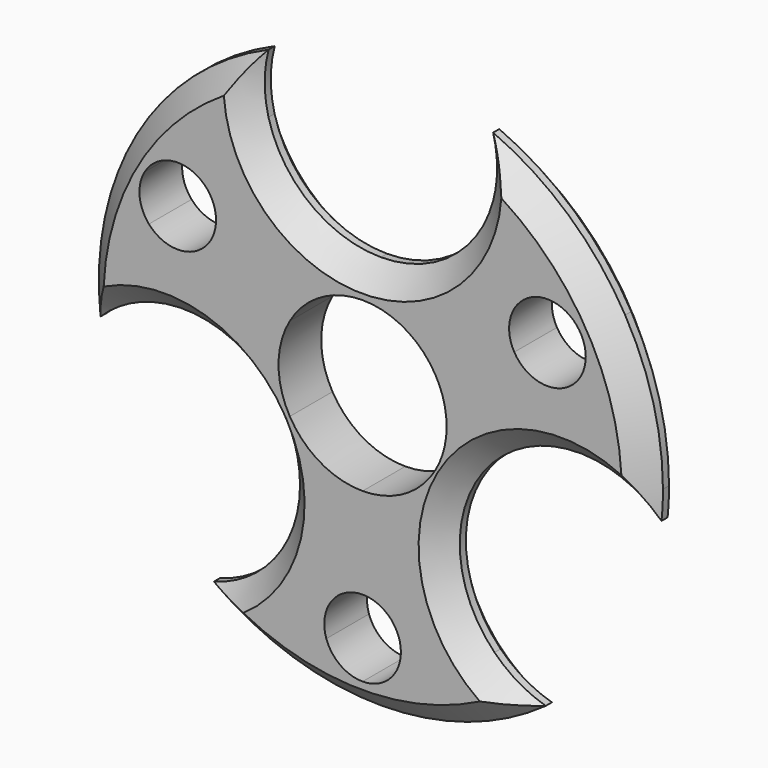
from build123d import *

# Parameters (mm, degrees)
F1_DEPTH     = 7
F2_T2_ANGLE  = 96.7405372454
F2_T4_ANGLE  = 266.8582437325
F2_T6_ANGLE  = 95.969109219
F2_T8_ANGLE  = 264.3512540772
F2_T10_ANGLE = 268.0965177518
F2_T12_ANGLE = 96.2209043171
F2_T14_ANGLE = 96.2209043171
F2_T16_ANGLE = 264.3512540772
F2_T18_ANGLE = 95.969109219
F2_T20_ANGLE = 266.8582437325
F2_T22_ANGLE = 96.7405372454
F2_T24_ANGLE = 268.0965177518


# Not quite as in the source:
# - a fillet or chamfer that OpenCascade refuses, or shapes differently, is made with other operations: its cross-section is extruded or revolved along the edge and cut away or added


with BuildPart() as f1:
    # F0 (on Front) → F1 (new body)
    with BuildSketch(Plane.XZ):
        with BuildLine():
            Line((-28.60048896, 16.5125), (-32.04293994, 18.5))
            ThreePointArc((-32.04293994, 18.5), (-36.2110940276, 7.5997808734), (-36.7769641036, -4.0564653732))
            ThreePointArc((-36.7769641036, -4.0564653732), (-33.6399342951, -1.6712337769), (-29.9995629467, -0.1619351868))
            ThreePointArc((-29.9995629467, -0.1619351868), (-29.5180509711, 5.3558068364), (-28.030388979, 10.6909912395))
            ThreePointArc((-28.030388979, 10.6909912395), (-29.2497876853, 13.5102449097), (-28.60048896, 16.5125))
        make_face()
        with BuildLine():
            ThreePointArc((-28.030388979, 10.6909912395), (-29.5180509711, 5.3558068364), (-29.9995629467, -0.1619351868))
            ThreePointArc((-29.9995629467, -0.1619351868), (-20.1170678219, -0.7895806962), (-12.6676409298, -7.3136659008))
            Line((-12.6676409298, -7.3136659008), (-9.5479300767, -5.5125))
            ThreePointArc((-9.5479300767, -5.5125), (-11.025, 0), (-9.5479300767, 5.5125))
            Line((-9.5479300767, 5.5125), (-19.8969336519, 11.4875))
            ThreePointArc((-19.8969336519, 11.4875), (-23.7589562157, 8.9989236207), (-28.030388979, 10.6909912395))
        make_face()
        with BuildLine():
            ThreePointArc((0, 14.7547752324), (-9.310283358, 17.9279039927), (-14.7448970108, 26.1263853631))
            ThreePointArc((-14.7448970108, 26.1263853631), (-19.3469694385, 22.9280346638), (-23.2738644946, 18.9295333141))
            ThreePointArc((-23.2738644946, 18.9295333141), (-20.3661071395, 17.1899858756), (-19.223711306, 14))
            ThreePointArc((-19.223711306, 14), (-19.3949340289, 12.6994342984), (-19.8969336519, 11.4875))
            Line((-19.8969336519, 11.4875), (-9.5479300767, 5.5125))
            ThreePointArc((-9.5479300767, 5.5125), (-5.5125, 9.5479300767), (0, 11.025))
            Line((0, 11.025), (0, 14.7547752324))
        make_face()
        with BuildLine():
            ThreePointArc((-14.7448970108, 26.1263853631), (-15.2451824532, 30.0359191128), (-14.726480194, 33.9430520298))
            ThreePointArc((-14.726480194, 33.9430520298), (-24.6265431784, 27.6140067915), (-32.04293994, 18.5))
            Line((-32.04293994, 18.5), (-28.60048896, 16.5125))
            ThreePointArc((-28.60048896, 16.5125), (-26.3251091458, 18.5759367359), (-23.2738644946, 18.9295333141))
            ThreePointArc((-23.2738644946, 18.9295333141), (-19.3469694385, 22.9280346638), (-14.7448970108, 26.1263853631))
        make_face()
        with BuildLine():
            ThreePointArc((19.8969336519, 11.4875), (19.6727745701, 16.0763978398), (23.2738644946, 18.9295333141))
            ThreePointArc((23.2738644946, 18.9295333141), (19.3469694385, 22.9280346638), (14.7448970108, 26.1263853631))
            ThreePointArc((14.7448970108, 26.1263853631), (9.310283358, 17.9279039927), (0, 14.7547752324))
            Line((0, 14.7547752324), (0, 11.025))
            ThreePointArc((0, 11.025), (5.5125, 9.5479300767), (9.5479300767, 5.5125))
            Line((9.5479300767, 5.5125), (19.8969336519, 11.4875))
        make_face()
        with BuildLine():
            Line((28.60048896, 16.5125), (32.04293994, 18.5))
            ThreePointArc((32.04293994, 18.5), (24.6265431784, 27.6140067915), (14.726480194, 33.9430520298))
            ThreePointArc((14.726480194, 33.9430520298), (15.1149822826, 31.9885142218), (15.2452247676, 30))
            ThreePointArc((15.2452247676, 30), (15.1196254471, 28.0471035473), (14.7448970108, 26.1263853631))
            ThreePointArc((14.7448970108, 26.1263853631), (19.3469694385, 22.9280346638), (23.2738644946, 18.9295333141))
            ThreePointArc((23.2738644946, 18.9295333141), (26.3251091458, 18.5759367359), (28.60048896, 16.5125))
        make_face()
        with BuildLine():
            ThreePointArc((36.8122346311, -3.7228190211), (36.9530288431, -1.8637755563), (37, 0))
            ThreePointArc((37, 0), (35.7392555727, 9.5763046688), (32.04293994, 18.5))
            Line((32.04293994, 18.5), (28.60048896, 16.5125))
            ThreePointArc((28.60048896, 16.5125), (29.1024885831, 15.3005657016), (29.273711306, 14))
            ThreePointArc((29.273711306, 14), (28.9526221952, 12.2325590968), (28.030388979, 10.6909912395))
            ThreePointArc((28.030388979, 10.6909912395), (29.4933804082, 5.4900375314), (29.9997945679, 0.1110219992))
            ThreePointArc((29.9997945679, 0.1110219992), (33.6494620505, -1.3733111503), (36.8122346311, -3.7228190211))
        make_face()
        with BuildLine():
            ThreePointArc((12.4392811828, -7.1818223394), (19.983625223, -0.5594336383), (29.9997945679, 0.1110219992))
            ThreePointArc((29.9997945679, 0.1110219992), (29.4933804082, 5.4900375314), (28.030388979, 10.6909912395))
            ThreePointArc((28.030388979, 10.6909912395), (23.7589562157, 8.9989236207), (19.8969336519, 11.4875))
            Line((19.8969336519, 11.4875), (9.5479300767, 5.5125))
            ThreePointArc((9.5479300767, 5.5125), (10.6493322348, 2.8534799723), (11.025, 0))
            ThreePointArc((11.025, 0), (10.6493322348, -2.8534799723), (9.5479300767, -5.5125))
            Line((9.5479300767, -5.5125), (12.4392811828, -7.1818223394))
        make_face()
        with BuildLine():
            ThreePointArc((4.7565244845, -29.6205245536), (9.9921782342, -28.2870354427), (14.9037494122, -26.0360952037))
            ThreePointArc((14.9037494122, -26.0360952037), (10.476296354, -17.0266102837), (12.4392811828, -7.1818223394))
            Line((12.4392811828, -7.1818223394), (9.5479300767, -5.5125))
            ThreePointArc((9.5479300767, -5.5125), (5.5125, -9.5479300767), (0, -11.025))
            Line((0, -11.025), (0, -22.975))
            ThreePointArc((0, -22.975), (3.5532115755, -24.4467884245), (5.025, -28))
            ThreePointArc((5.025, -28), (4.9574267788, -28.8213067227), (4.7565244845, -29.6205245536))
        make_face()
        with BuildLine():
            ThreePointArc((-10.6080939152, -15), (-11.7862202639, -20.9020258568), (-15.1400214589, -25.8994160209))
            ThreePointArc((-15.1400214589, -25.8994160209), (-10.1207607074, -28.2412854294), (-4.7565244845, -29.6205245536))
            ThreePointArc((-4.7565244845, -29.6205245536), (-4.0861816456, -25.0753214605), (0, -22.975))
            Line((0, -22.975), (0, -11.025))
            ThreePointArc((0, -11.025), (-5.5125, -9.5479300767), (-9.5479300767, -5.5125))
            Line((-9.5479300767, -5.5125), (-12.6676409298, -7.3136659008))
            ThreePointArc((-12.6676409298, -7.3136659008), (-11.1319048818, -11.0212606962), (-10.6080939152, -15))
        make_face()
        with BuildLine():
            ThreePointArc((-21.9014841146, -29.8215525011), (-11.5239437142, -35.1596177634), (0, -37))
            Line((0, -37), (0, -33.025))
            ThreePointArc((0, -33.025), (-2.9246785395, -32.0861816456), (-4.7565244845, -29.6205245536))
            ThreePointArc((-4.7565244845, -29.6205245536), (-10.1207607074, -28.2412854294), (-15.1400214589, -25.8994160209))
            ThreePointArc((-15.1400214589, -25.8994160209), (-18.267298054, -28.2974207927), (-21.9014841146, -29.8215525011))
        make_face()
        with BuildLine():
            ThreePointArc((0, -37), (11.3644165831, -35.2115043093), (21.6301731615, -30.0189208501))
            ThreePointArc((21.6301731615, -30.0189208501), (18.0140533687, -28.4546333842), (14.9037494122, -26.0360952037))
            ThreePointArc((14.9037494122, -26.0360952037), (9.9921782342, -28.2870354427), (4.7565244845, -29.6205245536))
            ThreePointArc((4.7565244845, -29.6205245536), (2.9246785395, -32.0861816456), (0, -33.025))
            Line((0, -33.025), (0, -37))
        make_face()
    extrude(amount=F1_DEPTH)

    # F2: chamfer of 3 on 12 edges, made by hand

    # F2_s1 → F2_t2 (revolve, cut)
    with BuildSketch(Plane(origin=(0, 0, 0), x_dir=(0, 1, 0), z_dir=(0.9799112872, 0, 0.199433872))):
        Polygon((-4, 37), (-7, 34), (-7, 37), align=None)
    revolve(axis=Axis((0, -7, 0), (0, -1, 0)), revolution_arc=F2_T2_ANGLE, mode=Mode.SUBTRACT)

    # F2_s3 → F2_t4 (revolve, cut)
    with BuildSketch(Plane(origin=(-6.2136111397, 0, -20.8819053013), x_dir=(0, 1, 0), z_dir=(-0.2852012416, 0, -0.9584676582))):
        Polygon((-4, -35.9963697961), (-7, -38.9963697961), (-7, -35.9963697961), align=None)
    revolve(axis=Axis((-25.9807621135, -7, -15), (0, 1, 0)), revolution_arc=F2_T4_ANGLE, mode=Mode.SUBTRACT)

    # F2_s5 → F2_t6 (revolve, cut)
    with BuildSketch(Plane(origin=(0, 0, 0), x_dir=(0, 1, 0), z_dir=(-0.6659555398, 0, 0.7459914336))):
        Polygon((-4, 37), (-7, 34), (-7, 37), align=None)
    revolve(axis=Axis((0, -7, 0), (0, -1, 0)), revolution_arc=F2_T6_ANGLE, mode=Mode.SUBTRACT)

    # F2_s7 → F2_t8 (revolve, cut)
    with BuildSketch(Plane(origin=(21.7325989573, 0, 4.6890781514), x_dir=(0, 1, 0), z_dir=(0.977505701, 0, 0.2109089959))):
        Polygon((-4, -35.7785172869), (-7, -38.7785172869), (-7, -35.7785172869), align=None)
    revolve(axis=Axis((25.9807621135, -7, -15), (0, 1, 0)), revolution_arc=F2_T8_ANGLE, mode=Mode.SUBTRACT)

    # F2_s9 → F2_t10 (revolve, cut)
    with BuildSketch(Plane(origin=(-14.9917229855, 0, 15.4982388241), x_dir=(0, 1, 0), z_dir=(-0.6952640068, 0, 0.718754451))):
        Polygon((-4, -36.1031449725), (-7, -39.1031449725), (-7, -36.1031449725), align=None)
    revolve(axis=Axis((0, -7, 30), (0, 1, 0)), revolution_arc=F2_T10_ANGLE, mode=Mode.SUBTRACT)

    # F2_s11 → F2_t12 (revolve, cut)
    with BuildSketch(Plane(origin=(0, 0, 0), x_dir=(0, 1, 0), z_dir=(-0.3044454567, 0, -0.9525297706))):
        Polygon((-4, 37), (-7, 34), (-7, 37), align=None)
    revolve(axis=Axis((0, -7, 0), (0, -1, 0)), revolution_arc=F2_T12_ANGLE, mode=Mode.SUBTRACT)

    # F2_s13 → F2_t14 (revolve, cut)
    with BuildSketch(Plane(origin=(0, 0, 0), x_dir=(0, 1, 0), z_dir=(-0.3044454567, 0, -0.9525297706))):
        Polygon((-3, 37), (0, 34), (0, 37), align=None)
    revolve(axis=Axis((0, 0, 0), (0, -1, 0)), revolution_arc=F2_T14_ANGLE, mode=Mode.SUBTRACT)

    # F2_s15 → F2_t16 (revolve, cut)
    with BuildSketch(Plane(origin=(21.7325989573, 0, 4.6890781514), x_dir=(0, 1, 0), z_dir=(0.977505701, 0, 0.2109089959))):
        Polygon((-3, -35.7785172869), (0, -38.7785172869), (0, -35.7785172869), align=None)
    revolve(axis=Axis((25.9807621135, 0, -15), (0, 1, 0)), revolution_arc=F2_T16_ANGLE, mode=Mode.SUBTRACT)

    # F2_s17 → F2_t18 (revolve, cut)
    with BuildSketch(Plane(origin=(0, 0, 0), x_dir=(0, 1, 0), z_dir=(-0.6659555398, 0, 0.7459914336))):
        Polygon((-3, 37), (0, 34), (0, 37), align=None)
    revolve(axis=Axis((0, 0, 0), (0, -1, 0)), revolution_arc=F2_T18_ANGLE, mode=Mode.SUBTRACT)

    # F2_s19 → F2_t20 (revolve, cut)
    with BuildSketch(Plane(origin=(-6.2136111397, 0, -20.8819053013), x_dir=(0, 1, 0), z_dir=(-0.2852012416, 0, -0.9584676582))):
        Polygon((-3, -35.9963697961), (0, -38.9963697961), (0, -35.9963697961), align=None)
    revolve(axis=Axis((-25.9807621135, 0, -15), (0, 1, 0)), revolution_arc=F2_T20_ANGLE, mode=Mode.SUBTRACT)

    # F2_s21 → F2_t22 (revolve, cut)
    with BuildSketch(Plane(origin=(0, 0, 0), x_dir=(0, 1, 0), z_dir=(0.9799112872, 0, 0.199433872))):
        Polygon((-3, 37), (0, 34), (0, 37), align=None)
    revolve(axis=Axis((0, 0, 0), (0, -1, 0)), revolution_arc=F2_T22_ANGLE, mode=Mode.SUBTRACT)

    # F2_s23 → F2_t24 (revolve, cut)
    with BuildSketch(Plane(origin=(-14.9917229855, 0, 15.4982388241), x_dir=(0, 1, 0), z_dir=(-0.6952640068, 0, 0.718754451))):
        Polygon((-3, -36.1031449725), (0, -39.1031449725), (0, -36.1031449725), align=None)
    revolve(axis=Axis((0, 0, 30), (0, 1, 0)), revolution_arc=F2_T24_ANGLE, mode=Mode.SUBTRACT)


solid = f1.part
